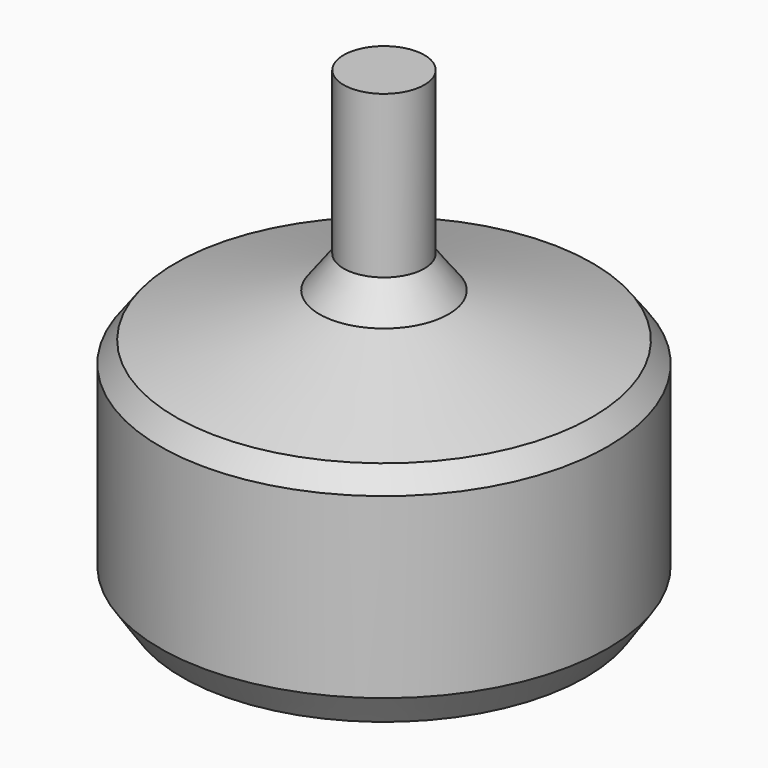
from build123d import *

# Parameters (mm, degrees)
F5_R       = 12.5
F6_R       = 13.85
F11_FACE_R = 13.85
F7_R       = 13.85
F12_FACE_R = 13.85
F9_R       = 4
F13_FACE_R = 4
F8_R       = 2.5
F14_FACE_R = 2.5
F10_R      = 2.5
F16_SIZE   = 1
F17_R      = 4.5
F18_DEPTH  = 2


with BuildPart() as f11:
    # F5 (on Top) → F11 section 0
    with BuildSketch(Plane.XY):
        Circle(F5_R)
    # F6 (on offset) → F11 section 1
    with BuildSketch(Plane.XY.offset(2)):
        Circle(F6_R)
    loft()

    # F11_face (on face) → F12 section 0
    with BuildSketch(Plane.XY.offset(2)):
        Circle(F11_FACE_R)
    # F7 (on offset) → F12 section 1
    with BuildSketch(Plane.XY.offset(14)):
        Circle(F7_R)
    loft()

    # F12_face (on face) → F13 section 0
    with BuildSketch(Plane.XY.offset(14)):
        Circle(F12_FACE_R)
    # F9 (on offset) → F13 section 1
    with BuildSketch(Plane.XY.offset(17)):
        Circle(F9_R)
    loft()

    # F13_face (on face) → F14 section 0
    with BuildSketch(Plane.XY.offset(17)):
        Circle(F13_FACE_R)
    # F8 (on offset) → F14 section 1
    with BuildSketch(Plane.XY.offset(19)):
        Circle(F8_R)
    loft()

    # F14_face (on face) → F15 section 0
    with BuildSketch(Plane.XY.offset(19)):
        Circle(F14_FACE_R)
    # F10 (on offset) → F15 section 1
    with BuildSketch(Plane.XY.offset(29)):
        Circle(F10_R)
    loft()

    # F16
    f16_edges = [f11.edges().sort_by_distance(p)[0] for p in [
        (-13.85, 0, 14),
    ]]
    chamfer(f16_edges, length=F16_SIZE)

    # F17 (on Top) → F18 (cut)
    with BuildSketch(Plane.XY):
        Circle(F17_R)
    extrude(amount=F18_DEPTH, mode=Mode.SUBTRACT)


solid = f11.part
